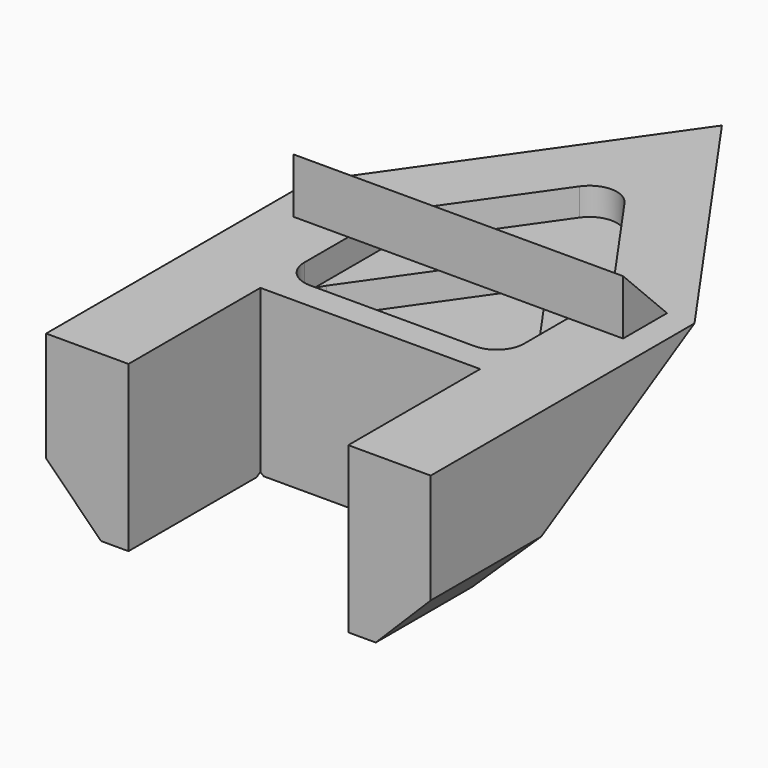
from build123d import *

# Parameters (mm, degrees)
F1_DEPTH    = 38.1
F2_T1_DEPTH = 273.4584537484
F2_T3_DEPTH = 273.4584537484
F3_SIZE     = 12.7
F5_DEPTH    = 6.35
F8_DEPTH    = 12.7
F9_DEPTH    = 38.1


# Not quite as in the source:
# - a fillet or chamfer that OpenCascade refuses, or shapes differently, is made with other operations: its cross-section is extruded or revolved along the edge and cut away or added


with BuildPart() as f1:
    # F0 (on Top) → F1 (new body)
    with BuildSketch(Plane.XY):
        Polygon((0, 63.4811788997), (-44.45, 0), (44.45, 0), align=None)
        Polygon((44.45, 0), (-44.45, 0), (-44.45, -76.2188211003), (-25.4, -76.2188211003), (-25.4, -38.1188211003), (25.4, -38.1188211003), (25.4, -76.2188211003), (44.45, -76.2188211003), align=None)
    extrude(amount=-F1_DEPTH)

    # F2: chamfer of 38.1 on 2 edges, made by hand

    # F2_s2 → F2_t1 (cut)
    with BuildSketch(Plane(origin=(70.8232650101, -101.1461047552, 0), x_dir=(0, 0, 1), z_dir=(-0.5735764364, 0.8191520443, 0))):
        Polygon((0, 36.4113083686), (-38.1, -1.6886916314), (-38.1, 36.4113083686), align=None)
    extrude(amount=F2_T1_DEPTH, mode=Mode.SUBTRACT)

    # F2_s4 → F2_t3 (cut)
    with BuildSketch(Plane(origin=(86.0260603809, 122.8579466609, 0), x_dir=(0, 0, 1), z_dir=(-0.5735764364, -0.8191520443, 0))):
        Polygon((0, 36.4113083686), (-38.1, -1.6886916314), (-38.1, 36.4113083686), align=None)
    extrude(amount=F2_T3_DEPTH, mode=Mode.SUBTRACT)

    # F3
    f3_edges = [f1.edges().sort_by_distance(p)[0] for p in [
        (44.45, -71.322072, -38.1),
        (-44.45, -71.322072, -38.1),
    ]]
    chamfer(f3_edges, length=F3_SIZE)

    # F4 (on Top) → F5 (cut)
    with BuildSketch(Plane.XY):
        with BuildLine():
            ThreePointArc((5.2016154812, 28.8462825899), (0, 31.5540722191), (-5.2016154812, 28.8462825899))
            Line((-5.2016154812, 28.8462825899), (-24.2516154812, 1.6400630614))
            ThreePointArc((-24.2516154812, 1.6400630614), (-25.1061026373, -0.0926654825), (-25.4, -2.0021473094))
            Line((-25.4, -2.0021473094), (-25.4, -25.4188211003))
            ThreePointArc((-25.4, -25.4188211003), (-23.5401280605, -29.9089491608), (-19.05, -31.7688211003))
            Line((-19.05, -31.7688211003), (0, -31.7688211003))
            Line((0, -31.7688211003), (19.05, -31.7688211003))
            ThreePointArc((19.05, -31.7688211003), (23.5401280605, -29.9089491608), (25.4, -25.4188211003))
            Line((25.4, -25.4188211003), (25.4, -2.0021473094))
            ThreePointArc((25.4, -2.0021473094), (25.1061026373, -0.0926654825), (24.2516154812, 1.6400630614))
            Line((24.2516154812, 1.6400630614), (5.2016154812, 28.8462825899))
        make_face()
    extrude(amount=-F5_DEPTH, mode=Mode.SUBTRACT)

    # F7 (on Top) → F8 (cut)
    with BuildSketch(Plane.XY):
        with BuildLine():
            Line((-19.05, -31.7688211003), (0, -31.7688211003))
            Line((0, -31.7688211003), (19.05, -31.7688211003))
            ThreePointArc((19.05, -31.7688211003), (23.5401280605, -29.9089491608), (25.4, -25.4188211003))
            Line((25.4, -25.4188211003), (25.4, -24.1439216138))
            ThreePointArc((25.4, -24.1439216138), (25.1061026373, -22.2344397869), (24.2516154812, -20.5017112429))
            Line((24.2516154812, -20.5017112429), (5.2016154812, 6.7045082855))
            ThreePointArc((5.2016154812, 6.7045082855), (0, 9.4122979147), (-5.2016154812, 6.7045082855))
            Line((-5.2016154812, 6.7045082855), (-24.2516154812, -20.5017112429))
            ThreePointArc((-24.2516154812, -20.5017112429), (-25.1061026373, -22.2344397869), (-25.4, -24.1439216138))
            Line((-25.4, -24.1439216138), (-25.4, -25.4188211003))
            ThreePointArc((-25.4, -25.4188211003), (-23.5401280605, -29.9089491608), (-19.05, -31.7688211003))
        make_face()
    extrude(amount=-F8_DEPTH, mode=Mode.SUBTRACT)

    # F6 (on Right) → F9 (join, symmetric)
    with BuildSketch(Plane.YZ):
        Polygon((-12.7, 12.7), (-12.7, 0), (0, 0), align=None)
    extrude(amount=F9_DEPTH, both=True)


solid = f1.part
